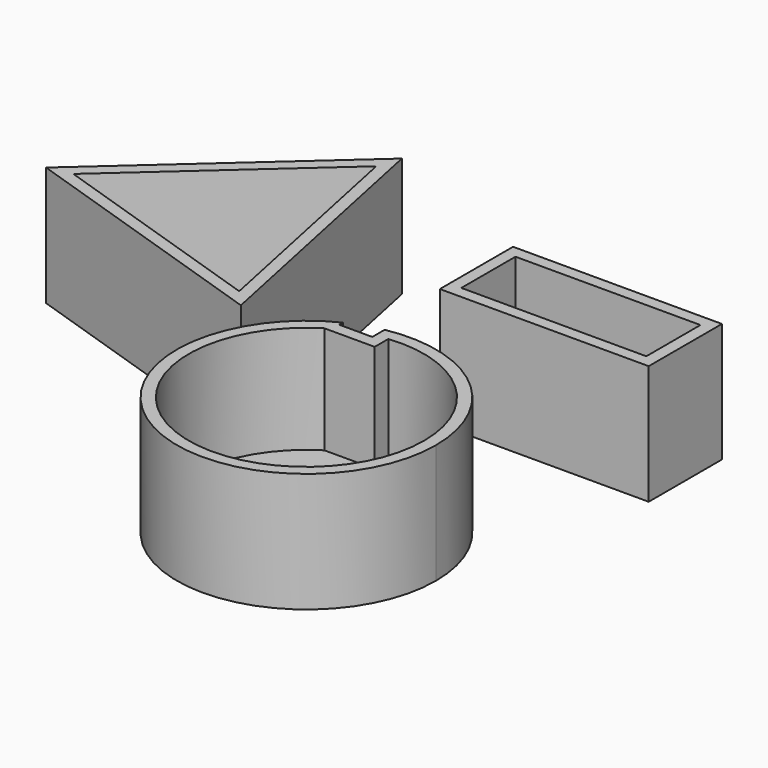
from build123d import *

# Parameters (mm, degrees)
F1_DEPTH      = 25.4
F0_W          = 44.4361274131
F0_H          = 19.472014159
F2_T          = -2.54
F2_2_T        = 2.54
F2_2_T3_DEPTH = 30.48
F2_3_T        = -2.54


# Not quite as in the source:
# - a shell that OpenCascade refuses in one call is made with other operations: the cavity is built on its own and cut out


with BuildPart() as f1:
    # F0 (on Top) → F1 (new body)
    with BuildSketch(Plane.XY):
        with BuildLine():
            Line((5.6169265881, 0.3058068698), (5.6169265881, -2.9956940562))
            Line((5.6169265881, -2.9956940562), (-1.3730227947, -2.9956940562))
            Line((-1.3730227947, -2.9956940562), (-1.3730227947, -1.9904286039))
            ThreePointArc((-1.3730227947, -1.9904286039), (-3.9889147019, -50.1545199575), (38.2132269141, -26.7963986844))
            ThreePointArc((38.2132269141, -26.7963986844), (28.2712658833, -5.6005952033), (5.6169265881, 0.3058068698))
        make_face()
    extrude(amount=F1_DEPTH)

    # F2#2: shell of thickness 2.54, made by hand


with BuildPart() as f1b:
    # F0 (on Top) → F1, piece 2 (new body)
    with BuildSketch(Plane.XY):
        Polygon((-18.5361797645, -7.750711828), (-30.6431320772, 50.1897106464), (-74.7675336897, 10.734571144), align=None)
    extrude(amount=F1_DEPTH)

    # F2
    f2_openings = [f1b.faces().sort_by_distance(p)[0] for p in [
        (-41.315615, 17.724523, 25.4),
    ]]
    offset(amount=F2_T, openings=f2_openings)


with BuildPart() as f1c:
    # F0 (on Top) → F1, piece 3 (new body)
    with BuildSketch(Plane.XY):
        with Locations((25.8378628641, 27.2108893842)):
            Rectangle(F0_W, F0_H)
    extrude(amount=F1_DEPTH)

    # F2#3
    f2_3_openings = [f1c.faces().sort_by_distance(p)[0] for p in [
        (25.837863, 27.210889, 25.4),
    ]]
    offset(amount=F2_3_T, openings=f2_3_openings)


with BuildPart() as f2_2_core1:
    # F2_2_t2: copy of F1
    add(f1.part)

    # the walls: a layer under each face that stays
    f2_2_faces = [f2_2_core1.faces().sort_by_distance(p)[0] for p in [
        (5.6169265881, -1.3449435932, 12.7),
        (2.1219518967, -2.9956940562, 12.7),
        (-1.3730227947, -2.4930613301, 12.7),
        (-3.9889147019, -50.1545199575, 12.7),
        (28.2712658833, -5.6005952033, 12.7),
        (10.6480075046, -26.7963986844, 0),
    ]]
    thicken(f2_2_faces, amount=-F2_2_T, mode=Mode.SUBTRACT)

    # F2_2_s4 → F2_2_t3 (cut)
    with BuildSketch(Plane.XY.offset(-2.54)):
        Polygon((5.5915265881, -2.9702940562), (8.1569265881, -2.9956940562), (8.1569265881, -5.5356940562), (5.6169265881, -5.5356940562), align=None)
        Polygon((-1.3476227947, -2.9702940562), (-1.3730227947, -5.5356940562), (-3.9130227947, -5.5356940562), (-3.9130227947, -2.9956940562), align=None)
    extrude(amount=F2_2_T3_DEPTH, mode=Mode.SUBTRACT)


with BuildPart() as f1_1:
    add(f1.part)

    # what is left inside the walls is the cavity
    f2_2_cavity = [f2_2_core1.part.solids().sort_by_distance(p)[0] for p in [
        (-1.503628, -48.644253, 17.78),
    ]]
    add(f2_2_cavity, mode=Mode.SUBTRACT)


solid = Compound([f1b.part, f1c.part, f1_1.part])
